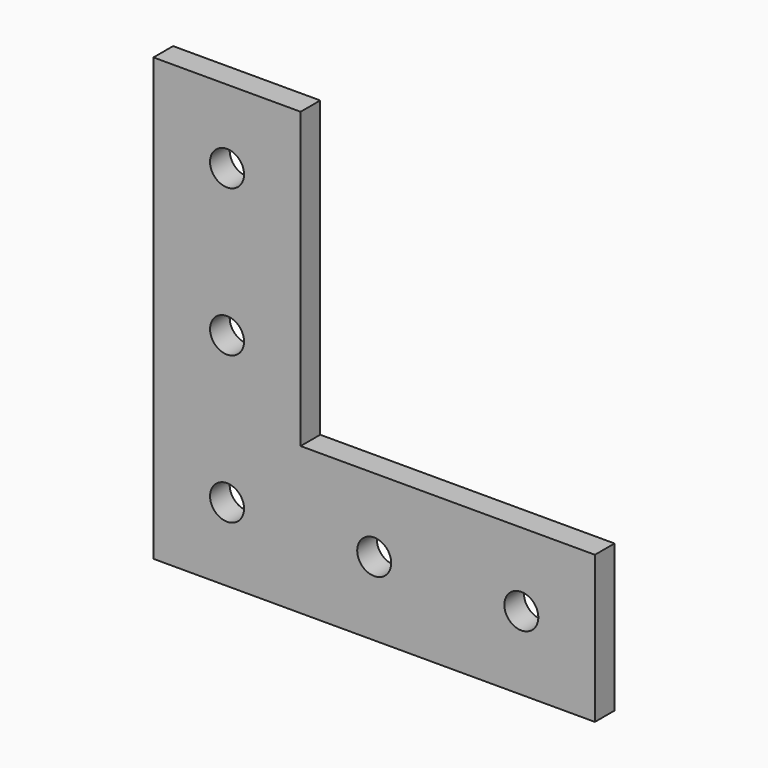
from build123d import *

# Parameters (mm, degrees)
F1_DEPTH = 6.35
F2_D     = 8.8


# Not quite as in the source:
# - a length typed as a fraction of an inch, garbled in the dataset ("3 / 203.2 mm" for 3/8 in), is restored


with BuildPart() as f1:
    # F0 (on Front) → F1 (new body)
    with BuildSketch(Plane.XZ):
        Polygon((0, 114.3), (0, 0), (114.3, 0), (114.3, 38.1), (38.1, 38.1), (38.1, 114.3), align=None)
    extrude(amount=-F1_DEPTH)

    # F2 (through all)
    with Locations(Plane.XZ):
        with Locations((19.05, 95.25), (19.05, 57.15), (19.05, 19.05), (57.15, 19.05), (95.25, 19.05)):
            Hole(F2_D / 2)


solid = f1.part
